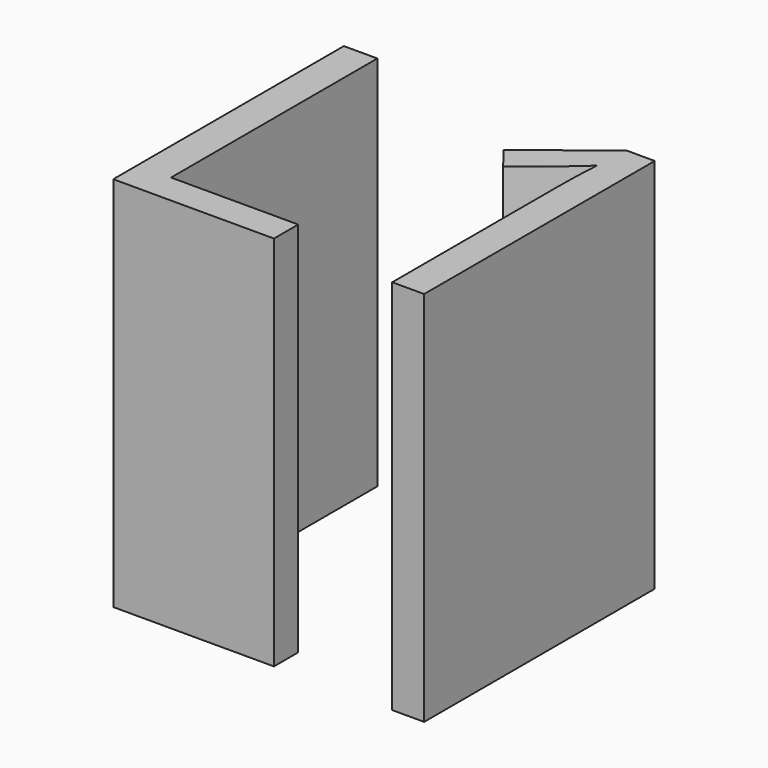
from build123d import *

# Parameters (mm, degrees)
F0_TEXT_SIZE = 10.7184726177
F1_DEPTH     = 10


# Not quite as in the source:
# - Text() gives the source's letters only with a copy of the font that has no kerning and outlines rounded to 1/6400 em; it was checked with that copy


with BuildPart() as f1:
    # F0 (on Top) → F1 (new body)
    with BuildSketch(Plane.XY):
        with Locations((-5, -3.8586501424)):
            Text('L1', F0_TEXT_SIZE, font='Open Sans', text_align=(TextAlign.LEFT, TextAlign.BOTTOM))
    extrude(amount=F1_DEPTH)


solid = f1.part
